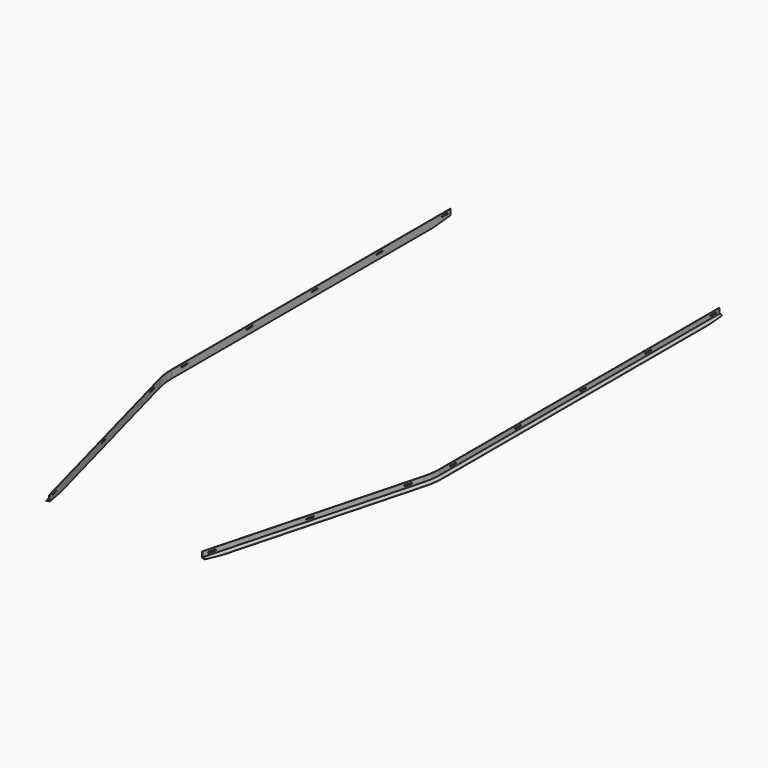
from build123d import *

# Parameters (mm, degrees)
F3_R        = 6.3
F4_T1_DEPTH = 972.9923861131
F4_T3_DEPTH = 1572.9923861131
F4_T6_ANGLE = 15
F5_W        = 35
F5_H        = 5
F6_DEPTH    = 25
F7_W        = 33.8074039201
F7_H        = 5
F8_DEPTH    = 25
F9_R        = 2.49999
F10_R       = 2.49999
F11_R       = 2.49999
F13_DEPTH   = 25
F15_DEPTH   = 25


# Not quite as in the source:
# - a fillet or chamfer that OpenCascade refuses, or shapes differently, is made with other operations: its cross-section is extruded or revolved along the edge and cut away or added
# - a fillet or chamfer is up to 0.001 mm smaller than in the source, because OpenCascade refuses the exact size


with BuildPart() as f2:
    # F2: sweep along a path in F1
    with BuildLine(Plane.XY) as f2_path:
        Line((0, 0), (0, -1560.5042507238))
        ThreePointArc((0, -1560.5042507238), (-2.5665415879, -1599.6621083898), (-10.2222521133, -1638.1499642545))
        Line((-10.2222521133, -1638.1499642545), (-258.8190451025, -2565.9258262891))
    # F0 (on Front) → F2 (sweep)
    with BuildSketch(Plane.XZ):
        with BuildLine():
            Line((0, 35), (0, 0))
            Line((0, 0), (1.5, 0))
            Line((1.5, 0), (4.5, 0))
            Line((4.5, 0), (4.5, 1.5))
            ThreePointArc((4.5, 1.5), (6.8588989435, 10.9085820594), (9.2177978871, 1.5))
            Line((9.2177978871, 1.5), (9.2177978871, 0))
            Line((9.2177978871, 0), (14, 0))
            Line((14, 0), (14, 12.5))
            Line((14, 12.5), (1.5, 12.5))
            Line((1.5, 12.5), (1.5, 35))
            Line((1.5, 35), (0, 35))
        make_face()
    sweep(path=f2_path.line)

    # F3
    f3_edges = [f2.edges().sort_by_distance(p)[0] for p in [
        (-120.997687, -2105.661362, 12.5),
        (14, -780.252125, 12.5),
        (11.313686, -1601.489475, 12.5),
    ]]
    fillet(f3_edges, radius=F3_R)

    # F4: fillet of radius 5 on 1 edges, made by hand

    # F4_s2 → F4_t1 (cut)
    with BuildSketch(Plane(origin=(-410.2222521133, -1530.9702872821, 0), x_dir=(0, 0, 1), z_dir=(-0.2588190451, -0.9659258263, 0))):
        with BuildLine():
            ThreePointArc((4.9952541557, -428.110472164), (1.5375807642, -426.7221884759), (0, -423.3282700511))
            Line((0, -423.3282700511), (0, -428.110472164))
            Line((0, -428.110472164), (4.9952541557, -428.110472164))
        make_face()
    extrude(amount=F4_T1_DEPTH, mode=Mode.SUBTRACT)

    # F4_s4 → F4_t3 (cut)
    with BuildSketch(Plane.XZ.offset(-12.4881353893)):
        with BuildLine():
            ThreePointArc((9.2177978871, 0), (12.6117163119, 1.5375807642), (14, 4.9952541557))
            Line((14, 4.9952541557), (14, 0))
            Line((14, 0), (9.2177978871, 0))
        make_face()
    extrude(amount=F4_T3_DEPTH, mode=Mode.SUBTRACT)

    # F4_s5 → F4_t6 (revolve, cut)
    with BuildSketch(Plane.XZ.offset(1560.5042507238)):
        with BuildLine():
            ThreePointArc((9.2177978871, 0), (12.6117163119, 1.5375807642), (14, 4.9952541557))
            Line((14, 4.9952541557), (14, 0))
            Line((14, 0), (9.2177978871, 0))
        make_face()
    revolve(axis=Axis((-300, -1560.5042507238, 0), (0, 0, -1)), revolution_arc=F4_T6_ANGLE, mode=Mode.SUBTRACT)

    # F5 (on face) → F6 (cut)
    with BuildSketch(Plane(origin=(401.4488887394, -107.5679055401, 0), x_dir=(0.2588190451, 0.9659258263, 0), z_dir=(0.9659258263, -0.2588190451, 0))):
        with Locations((-2502.9813220625, 23.5)):
            Rectangle(F5_W, F5_H)
        with Locations((-2077.9813220625, 23.5)):
            Rectangle(F5_W, F5_H)
        with Locations((-1652.9813220625, 23.5)):
            Rectangle(F5_W, F5_H)
    extrude(amount=-F6_DEPTH, mode=Mode.SUBTRACT)

    # F7 (on face) → F8 (cut)
    with BuildSketch(Plane.YZ.offset(1.5)):
        with Locations((-1488.6005487637, 23.5)):
            Rectangle(F7_W, F7_H)
        with Locations((-1124.7931448436, 23.5)):
            Rectangle(F7_W, F7_H)
        with Locations((-760.9857409235, 23.5)):
            Rectangle(F7_W, F7_H)
        with Locations((-397.1783370034, 23.5)):
            Rectangle(F7_W, F7_H)
        with Locations((-33.3709330832, 23.5)):
            Rectangle(F7_W, F7_H)
    extrude(amount=-F8_DEPTH, mode=Mode.SUBTRACT)

    # F9 (radius 2.5 in the source; OpenCascade refuses exactly that, so slightly less here)
    f9_edges = [f2.edges().sort_by_distance(p)[0] for p in [
        (-251.624125, -2541.971795, 26),
        (-251.624125, -2541.971795, 21),
        (-242.565458, -2508.164391, 26),
        (-242.565458, -2508.164391, 21),
    ]]
    fillet(f9_edges, radius=F9_R)

    # F10 (radius 2.5 in the source; OpenCascade refuses exactly that, so slightly less here)
    f10_edges = [f2.edges().sort_by_distance(p)[0] for p in [
        (-132.567364, -2097.645915, 21),
        (-132.567364, -2097.645915, 26),
        (-141.62603, -2131.453319, 21),
        (-141.62603, -2131.453319, 26),
        (-31.627936, -1720.934843, 21),
        (-31.627936, -1720.934843, 26),
        (-22.56927, -1687.127439, 21),
        (-22.56927, -1687.127439, 26),
        (0.75, -1471.696847, 21),
        (0.75, -1471.696847, 26),
        (0.75, -1505.504251, 21),
        (0.75, -1505.504251, 26),
        (0.75, -1141.696847, 21),
        (0.75, -1141.696847, 26),
        (0.75, -1107.889443, 21),
        (0.75, -1107.889443, 26),
    ]]
    fillet(f10_edges, radius=F10_R)

    # F11 (radius 2.5 in the source; OpenCascade refuses exactly that, so slightly less here)
    f11_edges = [f2.edges().sort_by_distance(p)[0] for p in [
        (0.75, -744.082039, 21),
        (0.75, -744.082039, 26),
        (0.75, -777.889443, 21),
        (0.75, -777.889443, 26),
        (0.75, -380.274635, 21),
        (0.75, -380.274635, 26),
        (0.75, -414.082039, 21),
        (0.75, -414.082039, 26),
        (0.75, -16.467231, 21),
        (0.75, -16.467231, 26),
        (0.75, -50.274635, 21),
        (0.75, -50.274635, 26),
    ]]
    fillet(f11_edges, radius=F11_R)

    # F12 (on face) → F13 (cut)
    with BuildSketch(Plane(origin=(400, -107.1796769724, 0), x_dir=(-0.2588190451, -0.9659258263, 0), z_dir=(-0.9659258263, 0.2588190451, 0))):
        Polygon((2445.4813220625, 0), (2545.4813220625, 0), (2545.4813220625, 9), align=None)
    extrude(amount=-F13_DEPTH, mode=Mode.SUBTRACT)

    # F14 (on face) → F15 (cut)
    with BuildSketch(Plane(origin=(0, 0, 0), x_dir=(0, -1, 0), z_dir=(-1, 0, 0))):
        Polygon((0, 9), (0, 0), (100, 0), align=None)
    extrude(amount=-F15_DEPTH, mode=Mode.SUBTRACT)


with BuildPart() as f17_1:
    # F17: instance of F2
    add(f2.part.mirror(Plane.YZ.offset(-600)))


solid = Compound([f2.part, f17_1.part])
